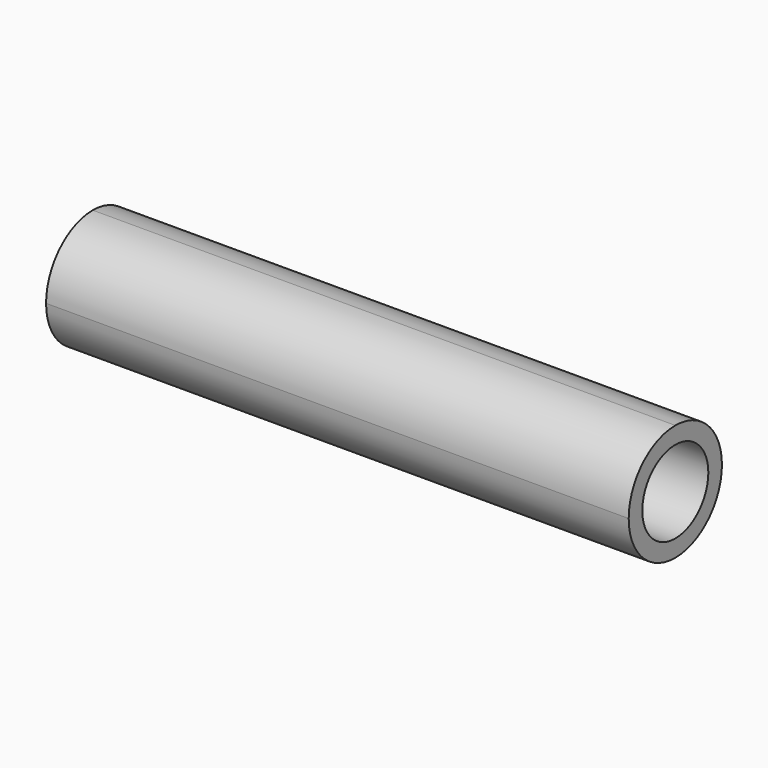
from build123d import *

# Parameters (mm, degrees)
F0_W     = 60
F0_H     = 12
F1_DEPTH = 12
F2_R     = 4.25
F4_DEPTH = 20
F3_R     = 4.25
F5_DEPTH = 20
F6_R     = 5.99999


# Not quite as in the source:
# - a fillet or chamfer is up to 0.001 mm smaller than in the source, because OpenCascade refuses the exact size


with BuildPart() as f1:
    # F0 (on Top) → F1 (new body)
    with BuildSketch(Plane.XY):
        Rectangle(F0_W, F0_H)
    extrude(amount=F1_DEPTH)

    # F2 (on face) → F4 (cut)
    with BuildSketch(Plane.YZ.offset(30)):
        with Locations((0, 6)):
            Circle(F2_R)
    extrude(amount=-F4_DEPTH, mode=Mode.SUBTRACT)

    # F3 (on face) → F5 (cut)
    with BuildSketch(Plane(origin=(-30, 0, 0), x_dir=(0, -1, 0), z_dir=(-1, 0, 0))):
        with Locations((0, 6)):
            Circle(F3_R)
    extrude(amount=-F5_DEPTH, mode=Mode.SUBTRACT)

    # F6 (radius 6 in the source; OpenCascade refuses exactly that, so slightly less here)
    f6_edges = [f1.edges().sort_by_distance(p)[0] for p in [
        (0, -6, 12),
        (0, -6, 0),
        (0, 6, 0),
        (0, 6, 12),
    ]]
    fillet(f6_edges, radius=F6_R)


solid = f1.part
